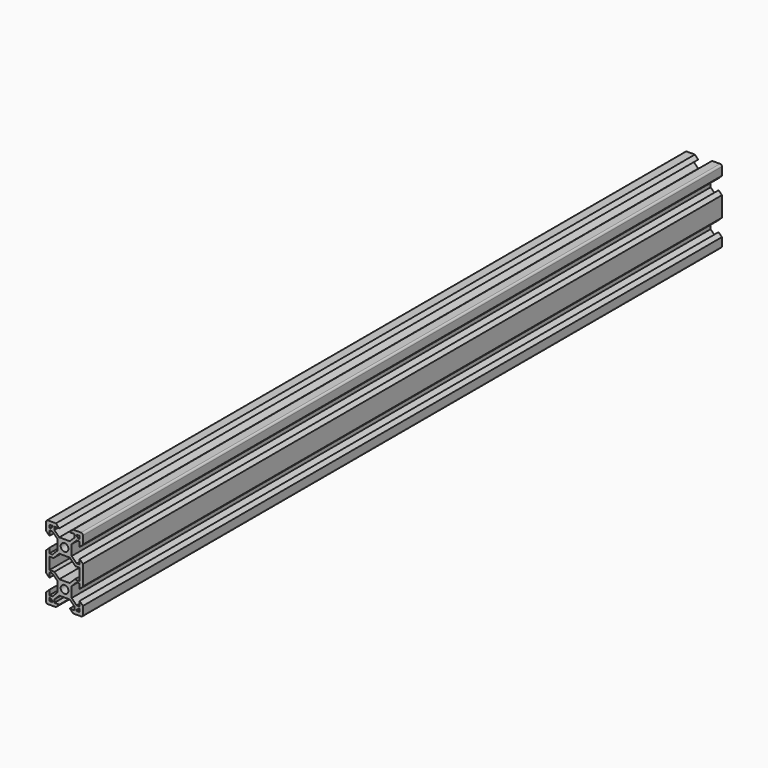
from build123d import *

# Parameters (mm, degrees)
F0_W             = 20
F0_H             = 20
F1_DEPTH         = 433
F2_R             = 2.1
F3_DEPTH         = 433.001
F4_R             = 1
F6_DEPTH         = 433.001
F6_COPIES3_COUNT = 2
F6_COPIES3_ANGLE = 90
F6_COPIES4_COUNT = 2
F6_COPIES4_ANGLE = 270
F6_COPIES6_COUNT = 2
F9_W             = 16.4
F9_H             = 6.8613203436
F10_DEPTH        = 433.001
F12_DEPTH        = 433


# Not quite as in the source:
# - a pattern or mirror of a feature is missing from the dataset's text; its kind, count and spacing are read off the source's solid


with BuildPart() as f1:
    # F0 (on Front) → F1 (new body)
    with BuildSketch(Plane.XZ):
        Rectangle(F0_W, F0_H)
    extrude(amount=F1_DEPTH)

    # F2 (on face) → F3 (cut, through all)
    with BuildSketch(Plane.XZ.offset(433)):
        Circle(F2_R)
    extrude(amount=-F3_DEPTH, mode=Mode.SUBTRACT)

    # F4
    f4_edges = [f1.edges().sort_by_distance(p)[0] for p in [
        (-10, -216.5, 10),
        (10, -216.5, 10),
    ]]
    fillet(f4_edges, radius=F4_R)

    # F5 (on face) → F6 (cut, through all)
    with BuildSketch(Plane.XZ.offset(433)):
        Polygon((0, 3.9006601718), (0, 10), (-2.84, 10), (-4.64, 10), (-2.84, 8.2), (-5.4993398282, 8.2), (-5.4993398282, 6.56), (-2.84, 3.9006601718), align=None)
        Polygon((-6.5693398282, 8.2), (-8.2, 8.2), (-7.0953059148, 7.0953059148), (-6.5693398282, 7.6212720014), align=None)
    f6 = extrude(amount=-F6_DEPTH, mode=Mode.SUBTRACT)

    # F6_copies: F6 across plane
    add(f6.mirror(Plane(origin=(0, 0, 0), x_dir=(-0.7071067812, 0, -0.7071067812), z_dir=(0.7071067812, 0, -0.7071067812))), mode=Mode.SUBTRACT)

    # F6_copies1: F6 across plane
    add(f6.mirror(Plane(origin=(0, 0, 0), x_dir=(0.7071067812, 0, -0.7071067812), z_dir=(-0.7071067812, 0, -0.7071067812))), mode=Mode.SUBTRACT)

    # F6_copies2: F6 across plane
    add(f6.mirror(Plane(origin=(0, 0, 0), x_dir=(0, 0, 1), z_dir=(1, 0, 0))), mode=Mode.SUBTRACT)

    # F6_copies3: F6 ×2 about axis
    f6_copies3_axis = Axis((0, 0, 0), (0, 1, 0))
    for i in range(1, F6_COPIES3_COUNT):
        add(f6.rotate(f6_copies3_axis, i * F6_COPIES3_ANGLE / (F6_COPIES3_COUNT - 1)), mode=Mode.SUBTRACT)

    # F6_copies4: F6 ×2 about axis
    f6_copies4_axis = Axis((0, 0, 0), (0, 1, 0))
    for i in range(1, F6_COPIES4_COUNT):
        add(f6.rotate(f6_copies4_axis, i * F6_COPIES4_ANGLE / (F6_COPIES4_COUNT - 1)), mode=Mode.SUBTRACT)

    # F6_copies5: F6 across plane
    add(f6.mirror(Plane(origin=(0, 0, 0), x_dir=(-1, 0, 0), z_dir=(0, 0, -1))), mode=Mode.SUBTRACT)

    # F6_copies6: F6 ×2 about axis
    f6_copies6_axis = Axis((0, 0, 0), (0, 1, 0))
    for i in range(1, F6_COPIES6_COUNT):
        add(f6.rotate(f6_copies6_axis, i * 360 / F6_COPIES6_COUNT), mode=Mode.SUBTRACT)

    # F8: F1 across face


with BuildPart() as f1_1:
    add(f1.part)
    add(f1.part.mirror(Plane(origin=(-7.32, -216.5, -10), x_dir=(1, 0, 0), z_dir=(0, 0, -1))))

    # F9 (on face) → F10 (cut, through all)
    with BuildSketch(Plane.XZ.offset(433)):
        with Locations((0, -10)):
            Rectangle(F9_W, F9_H)
    extrude(amount=-F10_DEPTH, mode=Mode.SUBTRACT)

    # F11 (on face) → F12 (join, through all)
    with BuildSketch(Plane.XZ.offset(433)):
        with BuildLine():
            ThreePointArc((-9, -10), (-9.7071067812, -9.7071067812), (-10, -9))
            Line((-10, -9), (-10, -11))
            ThreePointArc((-10, -11), (-9.7071067812, -10.2928932188), (-9, -10))
        make_face()
        with BuildLine():
            ThreePointArc((10, -9), (9.7071067812, -9.7071067812), (9, -10))
            ThreePointArc((9, -10), (9.7071067812, -10.2928932188), (10, -11))
            Line((10, -11), (10, -9))
        make_face()
        Polygon((5.9386796564, -6.9993398282), (8.2, -6.9993398282), (8.2, -6.5693398282), (5.5086796564, -6.5693398282), align=None)
        Polygon((-8.2, -6.5693398282), (-8.2, -6.9993398282), (-5.9386796564, -6.9993398282), (-5.5086796564, -6.5693398282), align=None)
    extrude(amount=-F12_DEPTH)


solid = f1_1.part
